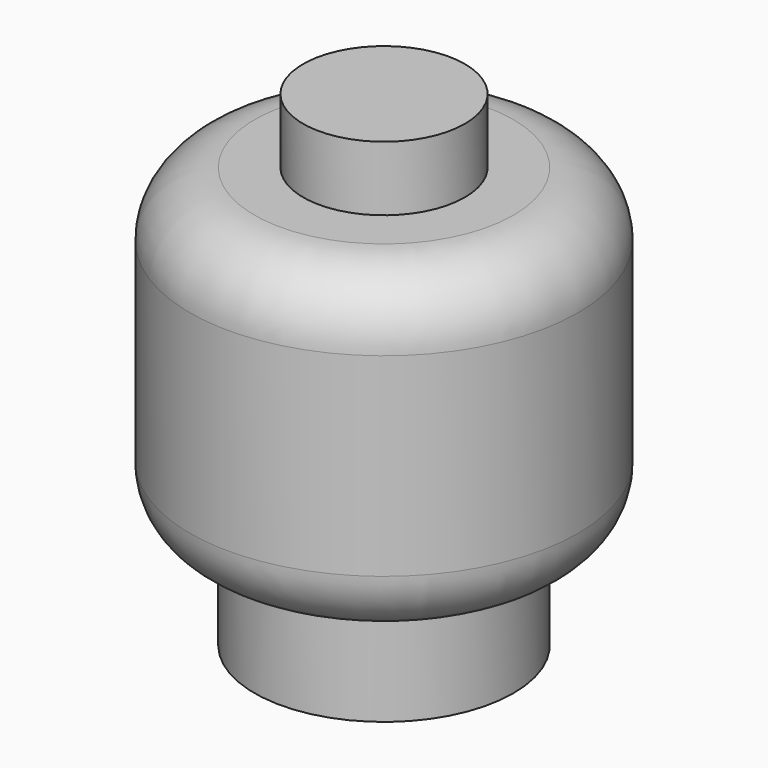
from build123d import *

# Parameters (mm, degrees)
F0_R     = 4
F1_DEPTH = 3
F2_R     = 6
F3_DEPTH = 10
F4_R     = 2.5
F5_DEPTH = 2
F6_R     = 1.99999
F7_R     = 2.5
F8_DEPTH = 8


# Not quite as in the source:
# - a fillet or chamfer is up to 0.001 mm smaller than in the source, because OpenCascade refuses the exact size


with BuildPart() as f1:
    # F0 (on Top) → F1 (new body)
    with BuildSketch(Plane.XY):
        Circle(F0_R)
    extrude(amount=F1_DEPTH)

    # F2 (on face) → F3 (join)
    with BuildSketch(Plane.XY.offset(3)):
        Circle(F2_R)
    extrude(amount=F3_DEPTH)

    # F4 (on face) → F5 (join)
    with BuildSketch(Plane.XY.offset(13)):
        Circle(F4_R)
    extrude(amount=F5_DEPTH)

    # F6 (radius 2 in the source; OpenCascade refuses exactly that, so slightly less here)
    f6_edges = [f1.edges().sort_by_distance(p)[0] for p in [
        (-6, 0, 13),
        (-6, 0, 3),
    ]]
    fillet(f6_edges, radius=F6_R)

    # F7 (on face) → F8 (cut)
    with BuildSketch(Plane(origin=(0, 0, 0), x_dir=(1, 0, 0), z_dir=(0, 0, -1))):
        Circle(F7_R)
    extrude(amount=-F8_DEPTH, mode=Mode.SUBTRACT)


solid = f1.part
